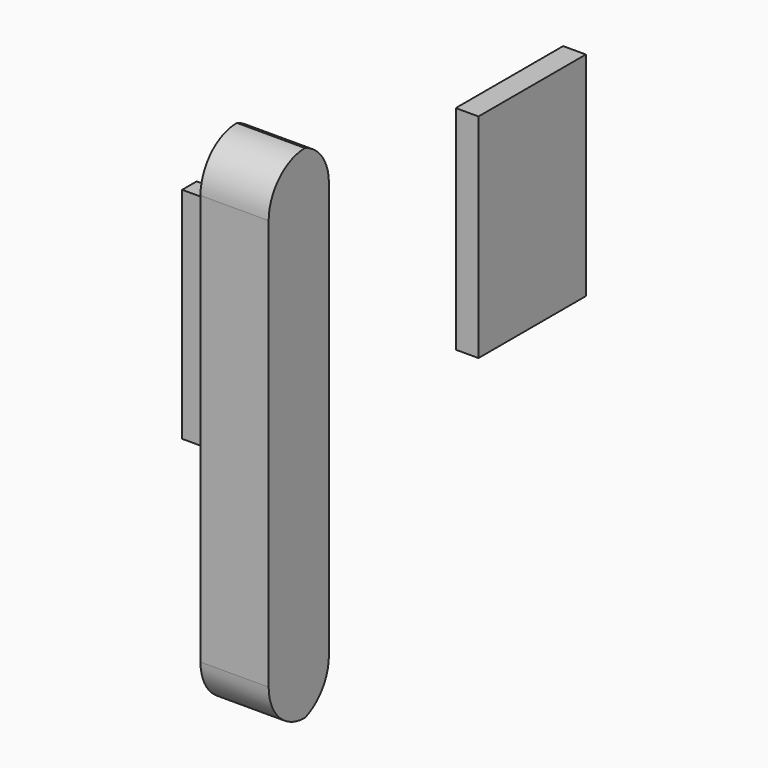
from build123d import *

# Parameters (mm, degrees)
F0_W        = 8.412479423
F0_H        = 56.0527183115
F1_DEPTH    = 7.62
F2_R        = 5.08
F3_T1_DEPTH = 31.4698280041
F4_R        = 5.08
F5_T1_DEPTH = 31.4698280041
F6_W        = 14.9961616844
F6_H        = 23.7744003534
F7_DEPTH    = 2.54
F8_W        = 8.7782405317
F8_H        = 24.5059225708
F9_DEPTH    = 1.016
F10_DEPTH   = 1.016


# Not quite as in the source:
# - a fillet or chamfer that OpenCascade refuses, or shapes differently, is made with other operations: its cross-section is extruded or revolved along the edge and cut away or added


with BuildPart() as f1:
    # F0 (on Right) → F1 (new body)
    with BuildSketch(Plane.YZ):
        with Locations((-4.2062397115, 28.0263591558)):
            Rectangle(F0_W, F0_H)
    extrude(amount=F1_DEPTH)

    # F2
    f2_edges = [f1.edges().sort_by_distance(p)[0] for p in [
        (3.81, -8.412479, 56.052718),
    ]]
    fillet(f2_edges, radius=F2_R)

    # F3: fillet of radius 5.08 on 1 edges, made by hand

    # F3_s2 → F3_t1 (cut)
    with BuildSketch(Plane.YZ.offset(-11.924914002)):
        with BuildLine():
            ThreePointArc((-3.332479423, 56.0527183115), (-0.9156390327, 54.1921336989), (0, 51.2827527107))
            Line((0, 51.2827527107), (0, 56.0527183115))
            Line((0, 56.0527183115), (-3.332479423, 56.0527183115))
        make_face()
    extrude(amount=F3_T1_DEPTH, mode=Mode.SUBTRACT)

    # F4
    f4_edges = [f1.edges().sort_by_distance(p)[0] for p in [
        (3.81, -8.412479, 0),
    ]]
    fillet(f4_edges, radius=F4_R)

    # F5: fillet of radius 5.08 on 1 edges, made by hand

    # F5_s2 → F5_t1 (cut)
    with BuildSketch(Plane.YZ.offset(-11.924914002)):
        with BuildLine():
            ThreePointArc((-3.332479423, 0), (-0.9156390327, 1.8605846126), (0, 4.7699656008))
            Line((0, 4.7699656008), (0, 0))
            Line((0, 0), (-3.332479423, 0))
        make_face()
    extrude(amount=F5_T1_DEPTH, mode=Mode.SUBTRACT)


with BuildPart() as f7:
    # F6 (on Right) → F7 (new body)
    with BuildSketch(Plane.YZ):
        with Locations((34.7471991554, 33.1927202642)):
            Rectangle(F6_W, F6_H)
    extrude(amount=F7_DEPTH)


with BuildPart() as f9:
    # F8 (on Front) → F9 (new body)
    with BuildSketch(Plane.XZ):
        with Locations((-4.3891202658, 33.0098411068)):
            Rectangle(F8_W, F8_H)
    extrude(amount=-F9_DEPTH)

    # F10 (add): a face of the model
    f10_faces = [f9.faces().sort_by_distance(p)[0] for p in [
        (-4.3891202658, 1.016, 33.0098411068),
    ]]
    extrude(f10_faces, amount=F10_DEPTH)


solid = Compound([f1.part, f7.part, f9.part])
